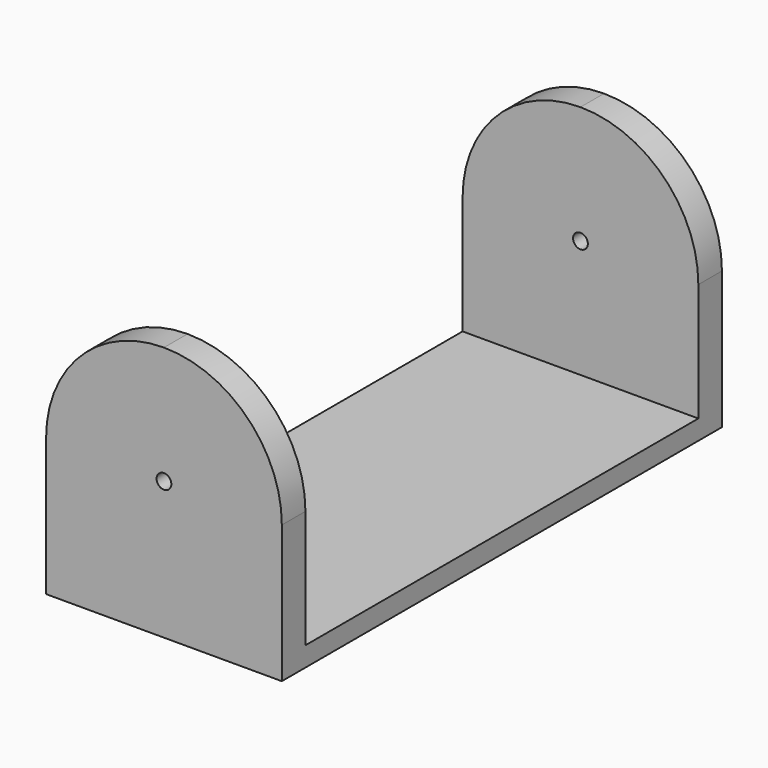
from build123d import *

# Parameters (mm, degrees)
F0_W     = 19.05
F0_H     = 152.4
F0_H_2   = 12.7
F0_W_2   = 317.5
F1_DEPTH = 152.4
F2_R     = 4.7625
F3_DEPTH = 406.4
F4_R     = 76.19999


# Not quite as in the source:
# - a fillet or chamfer is up to 0.001 mm smaller than in the source, because OpenCascade refuses the exact size


with BuildPart() as f1:
    # F0 (on Right) → F1 (new body)
    with BuildSketch(Plane.YZ):
        with Locations((9.525, 88.9)):
            Rectangle(F0_W, F0_H)
        with Locations((9.525, 6.35)):
            Rectangle(F0_W, F0_H_2)
        with Locations((177.8, 6.35)):
            Rectangle(F0_W_2, F0_H_2)
        with Locations((346.075, 88.9)):
            Rectangle(F0_W, F0_H)
        with Locations((346.075, 6.35)):
            Rectangle(F0_W, F0_H_2)
    extrude(amount=F1_DEPTH)

    # F2 (on Front) → F3 (cut)
    with BuildSketch(Plane.XZ):
        with Locations((76.2, 88.9)):
            Circle(F2_R)
    extrude(amount=-F3_DEPTH, mode=Mode.SUBTRACT)

    # F4 (radius 76.2 in the source; OpenCascade refuses exactly that, so slightly less here)
    f4_edges = [f1.edges().sort_by_distance(p)[0] for p in [
        (152.4, 346.075, 165.1),
        (152.4, 9.525, 165.1),
        (0, 9.525, 165.1),
        (0, 346.075, 165.1),
    ]]
    fillet(f4_edges, radius=F4_R)


solid = f1.part
